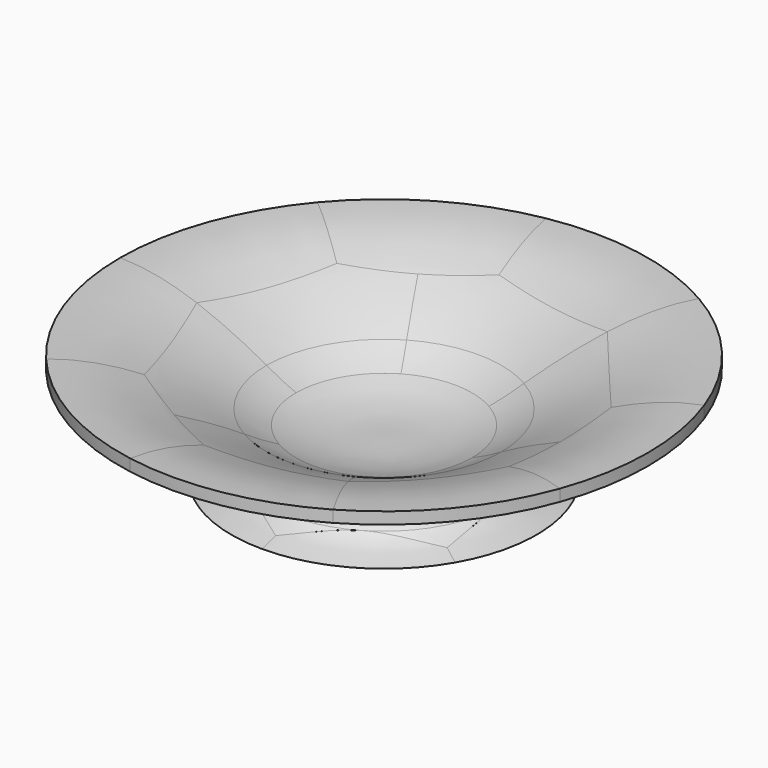
from build123d import *

# Parameters (mm, degrees)
F1_DEPTH  = 20.32
F2_DEPTH  = 20.32
F3_DEPTH  = 20.32
F6_DEPTH  = 6.35
F7_DEPTH  = 6.35
F8_ANGLE  = 60
F9_ANGLE  = 120
F10_ANGLE = -120
F12_DEPTH = 20.32
F14_ANGLE = 30
F19_W     = 304.8
F19_H     = 304.8
F20_DEPTH = 46.99


with BuildPart() as f1:
    # F0 (on Top) → F1 (new body)
    with BuildSketch(Plane.XY):
        Polygon((-14.0811908549, 79.8584016939), (-21.1217862823, 119.7876025409), (-93.1782137177, 78.1858047642), (-62.1188091451, 52.1238698428), (-38.1, 65.9911357684), align=None)
    extrude(amount=F1_DEPTH)


with BuildPart() as f1b:
    # F0 (on Top) → F1, piece 2 (new body)
    with BuildSketch(Plane.XY):
        Polygon((76.2, 27.7345318511), (114.3, 41.6017977766), (60.817759697, 105.3394497977), (40.5451731313, 70.2262998651), align=None)
    extrude(amount=F1_DEPTH)


with BuildPart() as f2:
    # F0 (on Top) → F2 (new body)
    with BuildSketch(Plane.XY):
        Polygon((-38.1, 65.9911357684), (-62.1188091451, 52.1238698428), (-81.0903462627, 0), (-48.2307597995, 0), (-24.1153798997, 41.7690632302), align=None)
    extrude(amount=F2_DEPTH)


with BuildPart() as f2b:
    # F0 (on Top) → F2, piece 2 (new body)
    with BuildSketch(Plane.XY):
        Polygon((40.5451731313, 70.2262998651), (60.817759697, 105.3394497977), (-21.1217862823, 119.7876025409), (-14.0811908549, 79.8584016939), align=None)
    extrude(amount=F2_DEPTH)


with BuildPart() as f3:
    # F0 (on Top) → F3 (new body)
    with BuildSketch(Plane.XY):
        Polygon((24.1153798997, 41.7690632302), (40.5451731313, 70.2262998651), (-14.0811908549, 79.8584016939), (-38.1, 65.9911357684), (-24.1153798997, 41.7690632302), align=None)
    extrude(amount=F3_DEPTH)


with BuildPart() as f6:
    # F5 (on Top) → F6 (new body)
    with BuildSketch(Plane.XY):
        Polygon((38.1, -65.9911357684), (76.2, 0), (38.1, 0), (19.05, -32.9955678842), align=None)
    extrude(amount=-F6_DEPTH)


with BuildPart() as f7:
    # F5 (on Top) → F7 (new body)
    with BuildSketch(Plane.XY):
        Polygon((38.1, 0), (76.2, 0), (38.1, 65.9911357684), (19.05, 32.9955678842), align=None)
    extrude(amount=-F7_DEPTH)


with BuildPart() as f6_1:
    # F8: moved
    add(f6.part.rotate(Axis((0, 0, 57.15), (0, 0, 1)), F8_ANGLE))


with BuildPart() as f7_1:
    # F8: moved
    add(f7.part.rotate(Axis((0, 0, 57.15), (0, 0, 1)), F8_ANGLE))


with BuildPart() as f9_1:
    # F9: copy of F2
    add(f2.part.rotate(Axis((0, 0, 57.15), (0, 0, 1)), F9_ANGLE))


with BuildPart() as f9_2:
    # F9: copy of F1b
    add(f1b.part.rotate(Axis((0, 0, 57.15), (0, 0, 1)), F9_ANGLE))


with BuildPart() as f9_3:
    # F9: copy of F3
    add(f3.part.rotate(Axis((0, 0, 57.15), (0, 0, 1)), F9_ANGLE))


with BuildPart() as f9_4:
    # F9: copy of F2b
    add(f2b.part.rotate(Axis((0, 0, 57.15), (0, 0, 1)), F9_ANGLE))


with BuildPart() as f9_5:
    # F9: copy of F1
    add(f1.part.rotate(Axis((0, 0, 57.15), (0, 0, 1)), F9_ANGLE))


with BuildPart() as f9_6:
    # F9: copy of F6
    add(f6_1.part.rotate(Axis((0, 0, 57.15), (0, 0, 1)), F9_ANGLE))


with BuildPart() as f9_7:
    # F9: copy of F7
    add(f7_1.part.rotate(Axis((0, 0, 57.15), (0, 0, 1)), F9_ANGLE))


with BuildPart() as f10_1:
    # F10: copy of F2b
    add(f2b.part.rotate(Axis((0, 0, 57.15), (0, 0, 1)), F10_ANGLE))


with BuildPart() as f10_2:
    # F10: copy of F3
    add(f3.part.rotate(Axis((0, 0, 57.15), (0, 0, 1)), F10_ANGLE))


with BuildPart() as f10_3:
    # F10: copy of F1
    add(f1.part.rotate(Axis((0, 0, 57.15), (0, 0, 1)), F10_ANGLE))


with BuildPart() as f10_4:
    # F10: copy of F2
    add(f2.part.rotate(Axis((0, 0, 57.15), (0, 0, 1)), F10_ANGLE))


with BuildPart() as f10_5:
    # F10: copy of F1b
    add(f1b.part.rotate(Axis((0, 0, 57.15), (0, 0, 1)), F10_ANGLE))


with BuildPart() as f10_6:
    # F10: copy of F6
    add(f6_1.part.rotate(Axis((0, 0, 57.15), (0, 0, 1)), F10_ANGLE))


with BuildPart() as f10_7:
    # F10: copy of F7
    add(f7_1.part.rotate(Axis((0, 0, 57.15), (0, 0, 1)), F10_ANGLE))


with BuildPart() as f12:
    # F11 (on face) → F12 (new body)
    with BuildSketch(Plane(origin=(0, 0, -6.35), x_dir=(1, 0, 0), z_dir=(0, 0, -1))):
        Polygon((50.8, -29.3293936748), (50.8, 29.3293936748), (0, 58.6587873497), (-50.8, 29.3293936748), (-50.8, -29.3293936748), (0, -58.6587873497), align=None)
    extrude(amount=F12_DEPTH)


with BuildPart() as f13_1:
    # F13: copy of F9_7
    add(f9_7.part.moved(Location((0, 0, -20.32))))


with BuildPart() as f13_2:
    # F13: copy of F9_6
    add(f9_6.part.moved(Location((0, 0, -20.32))))


with BuildPart() as f13_3:
    # F13: copy of F7
    add(f7_1.part.moved(Location((0, 0, -20.32))))


with BuildPart() as f13_4:
    # F13: copy of F6
    add(f6_1.part.moved(Location((0, 0, -20.32))))


with BuildPart() as f13_5:
    # F13: copy of F10_7
    add(f10_7.part.moved(Location((0, 0, -20.32))))


with BuildPart() as f13_6:
    # F13: copy of F10_6
    add(f10_6.part.moved(Location((0, 0, -20.32))))


with BuildPart() as f13_2_1:
    # F14: moved
    add(f13_2.part.rotate(Axis((0, 0, 57.15), (0, 0, 1)), F14_ANGLE))

    # F15: cut F12
    add(f12.part, mode=Mode.SUBTRACT)


with BuildPart() as f13_1_1:
    # F14: moved
    add(f13_1.part.rotate(Axis((0, 0, 57.15), (0, 0, 1)), F14_ANGLE))

    # F15: cut F12
    add(f12.part, mode=Mode.SUBTRACT)


with BuildPart() as f13_6_1:
    # F14: moved
    add(f13_6.part.rotate(Axis((0, 0, 57.15), (0, 0, 1)), F14_ANGLE))

    # F15: cut F12
    add(f12.part, mode=Mode.SUBTRACT)


with BuildPart() as f13_5_1:
    # F14: moved
    add(f13_5.part.rotate(Axis((0, 0, 57.15), (0, 0, 1)), F14_ANGLE))

    # F15: cut F12
    add(f12.part, mode=Mode.SUBTRACT)


with BuildPart() as f13_4_1:
    # F14: moved
    add(f13_4.part.rotate(Axis((0, 0, 57.15), (0, 0, 1)), F14_ANGLE))

    # F15: cut F12
    add(f12.part, mode=Mode.SUBTRACT)


with BuildPart() as f13_3_1:
    # F14: moved
    add(f13_3.part.rotate(Axis((0, 0, 57.15), (0, 0, 1)), F14_ANGLE))

    # F15: cut F12
    add(f12.part, mode=Mode.SUBTRACT)


with BuildPart() as f17:
    # F16 (on Right) → F17 (revolve)
    with BuildSketch(Plane.YZ):
        with BuildLine():
            add(Edge.make_bspline(
                [(-50.8, -20.32), (-49.0910434922, -18.3663345587), (-45.5553338467, -14.2749399627), (-49.9673850897, -4.4302862483), (-71.717735148, 4.6770569656), (-85.7510098211, 10.8503529448), (-103.4136962789, 15.0270716516), (-114.3, 15.24)],
                knots=[0, 0, 0, 0, 0.1354114311, 0.2843399499, 0.5254369108, 0.7289098909, 1, 1, 1, 1], degree=3))
            add(Edge.make_bspline(
                [(-50.8, -20.32), (-54.5365512371, -23.5419198871), (-59.902433306, -25.1491069794), (-66.04, -26.67)],
                knots=[0, 0, 0, 0, 16.51, 16.51, 16.51, 16.51], degree=3))
            Line((-66.04, -26.67), (0, -26.67))
            Line((0, -26.67), (0, -11.43))
            add(Edge.make_bspline(
                [(-114.3, 20.32), (-97.4674538559, 20.32), (-72.0181886042, 11.1394515548), (-51.0990109439, 0.3385451121), (-38.6481329844, -6.9737998953), (-19.5417697396, -11.5357841499), (-10.0679981986, -11.5973343434), (0, -11.43)],
                knots=[0, 0, 0, 0, 0.2781641942, 0.4763795266, 0.6335726516, 0.8086602438, 1, 1, 1, 1], degree=3))
            Line((-114.3, 20.32), (-114.3, 15.24))
        make_face()
    revolve(axis=Axis((0, 0, 57.15), (0, 0, 1)))


with BuildPart() as f17_1:
    # F18: moved
    add(f17.part.moved(Location((0, 304.8, 0))))


with BuildPart() as f20:
    # F19 (on face) → F20 (new body)
    with BuildSketch(Plane(origin=(0, 0, -26.67), x_dir=(1, 0, 0), z_dir=(0, 0, -1))):
        with Locations((0, -3.4923499916)):
            Rectangle(F19_W, F19_H)
    extrude(amount=-F20_DEPTH)


with BuildPart() as f20_1:
    # F21: moved
    add(f20.part.moved(Location((0, 304.8, 0))))

    # F22: cut F17
    add(f17_1.part, mode=Mode.SUBTRACT)


with BuildPart() as f20_2:
    # F23: moved
    add(f20_1.part.moved(Location((0, -304.8, 0))))


with BuildPart() as f1_1:
    add(f1.part)

    # F24: cut F20
    add(f20_2.part, mode=Mode.SUBTRACT)


with BuildPart() as f13_5_2:
    add(f13_5_1.part)

    # F24: cut F20
    add(f20_2.part, mode=Mode.SUBTRACT)


with BuildPart() as f13_2_2:
    add(f13_2_1.part)

    # F24: cut F20
    add(f20_2.part, mode=Mode.SUBTRACT)


with BuildPart() as f13_1_2:
    add(f13_1_1.part)

    # F24: cut F20
    add(f20_2.part, mode=Mode.SUBTRACT)


with BuildPart() as f13_6_2:
    add(f13_6_1.part)

    # F24: cut F20
    add(f20_2.part, mode=Mode.SUBTRACT)


with BuildPart() as f13_3_2:
    add(f13_3_1.part)

    # F24: cut F20
    add(f20_2.part, mode=Mode.SUBTRACT)


with BuildPart() as f3_1:
    add(f3.part)

    # F24: cut F20
    add(f20_2.part, mode=Mode.SUBTRACT)


with BuildPart() as f6_2:
    add(f6_1.part)

    # F24: cut F20
    add(f20_2.part, mode=Mode.SUBTRACT)


with BuildPart() as f7_2:
    add(f7_1.part)

    # F24: cut F20
    add(f20_2.part, mode=Mode.SUBTRACT)


with BuildPart() as f9_5_1:
    add(f9_5.part)

    # F24: cut F20
    add(f20_2.part, mode=Mode.SUBTRACT)


with BuildPart() as f9_2_1:
    add(f9_2.part)

    # F24: cut F20
    add(f20_2.part, mode=Mode.SUBTRACT)


with BuildPart() as f9_4_1:
    add(f9_4.part)

    # F24: cut F20
    add(f20_2.part, mode=Mode.SUBTRACT)


with BuildPart() as f9_1_1:
    add(f9_1.part)

    # F24: cut F20
    add(f20_2.part, mode=Mode.SUBTRACT)


with BuildPart() as f9_3_1:
    add(f9_3.part)

    # F24: cut F20
    add(f20_2.part, mode=Mode.SUBTRACT)


with BuildPart() as f9_6_1:
    add(f9_6.part)

    # F24: cut F20
    add(f20_2.part, mode=Mode.SUBTRACT)


with BuildPart() as f9_7_1:
    add(f9_7.part)

    # F24: cut F20
    add(f20_2.part, mode=Mode.SUBTRACT)


with BuildPart() as f10_3_1:
    add(f10_3.part)

    # F24: cut F20
    add(f20_2.part, mode=Mode.SUBTRACT)


with BuildPart() as f10_5_1:
    add(f10_5.part)

    # F24: cut F20
    add(f20_2.part, mode=Mode.SUBTRACT)


with BuildPart() as f10_1_1:
    add(f10_1.part)

    # F24: cut F20
    add(f20_2.part, mode=Mode.SUBTRACT)


with BuildPart() as f10_4_1:
    add(f10_4.part)

    # F24: cut F20
    add(f20_2.part, mode=Mode.SUBTRACT)


with BuildPart() as f10_2_1:
    add(f10_2.part)

    # F24: cut F20
    add(f20_2.part, mode=Mode.SUBTRACT)


with BuildPart() as f10_6_1:
    add(f10_6.part)

    # F24: cut F20
    add(f20_2.part, mode=Mode.SUBTRACT)


with BuildPart() as f10_7_1:
    add(f10_7.part)

    # F24: cut F20
    add(f20_2.part, mode=Mode.SUBTRACT)


with BuildPart() as f12_1:
    add(f12.part)

    # F24: cut F20
    add(f20_2.part, mode=Mode.SUBTRACT)


with BuildPart() as f13_4_2:
    add(f13_4_1.part)

    # F24: cut F20
    add(f20_2.part, mode=Mode.SUBTRACT)


with BuildPart() as f1b_1:
    add(f1b.part)

    # F24: cut F20
    add(f20_2.part, mode=Mode.SUBTRACT)


with BuildPart() as f2b_1:
    add(f2b.part)

    # F24: cut F20
    add(f20_2.part, mode=Mode.SUBTRACT)


with BuildPart() as f2_1:
    add(f2.part)

    # F24: cut F20
    add(f20_2.part, mode=Mode.SUBTRACT)


solid = Compound([f1_1.part, f13_5_2.part, f13_2_2.part, f13_1_2.part, f13_6_2.part, f13_3_2.part, f3_1.part, f6_2.part, f7_2.part, f9_5_1.part, f9_2_1.part, f9_4_1.part, f9_1_1.part, f9_3_1.part, f9_6_1.part, f9_7_1.part, f10_3_1.part, f10_5_1.part, f10_1_1.part, f10_4_1.part, f10_2_1.part, f10_6_1.part, f10_7_1.part, f12_1.part, f13_4_2.part, f1b_1.part, f2b_1.part, f2_1.part])
